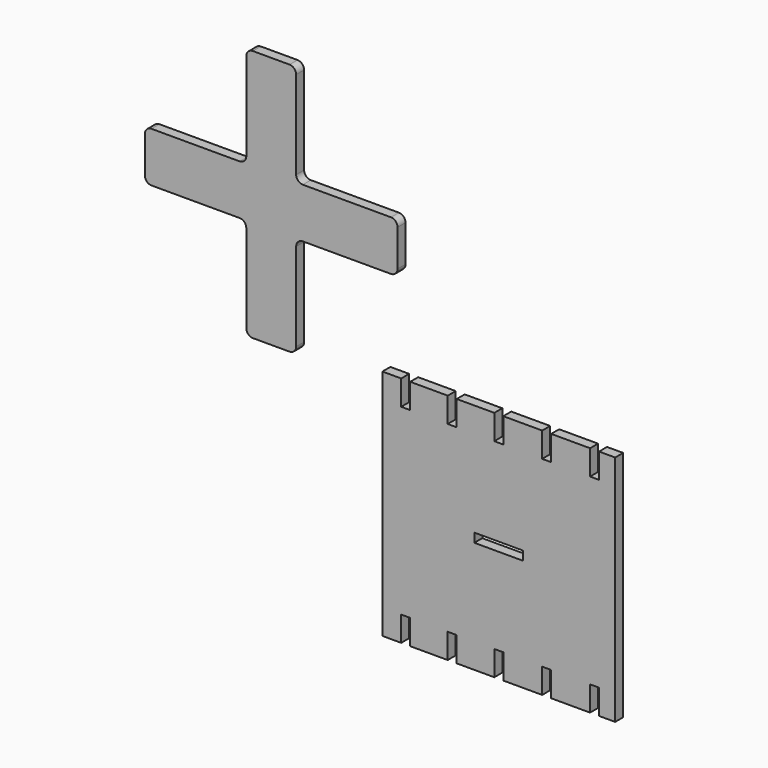
from build123d import *

# Parameters (mm, degrees)
F1_DEPTH = 3
F2_W     = 14.7
F2_H     = 2.7
F3_DEPTH = 3


# Not quite as in the source:
# - ends of sketch curves that miss each other by under 0.0002 mm in the source are joined


with BuildPart() as f1:
    # F0 (on Front) → F1 (new body)
    with BuildSketch(Plane.XZ):
        with BuildLine():
            ThreePointArc((-56.8837374449, 13.9543364197), (-56.2979510073, 12.5401228573), (-54.8837374449, 11.9543364197))
            Line((-54.8837374449, 11.9543364197), (-43.8837374449, 11.9543364197))
            ThreePointArc((-43.8837374449, 11.9543364197), (-42.4695238825, 12.5401228573), (-41.8837374449, 13.9543364197))
            Line((-41.8837374449, 13.9543364197), (-41.8837374449, 40.4543364197))
            ThreePointArc((-41.8837374449, 40.4543364197), (-41.2979510073, 41.8685499821), (-39.8837374449, 42.4543364197))
            Line((-39.8837374449, 42.4543364197), (-13.3837374449, 42.4543364197))
            ThreePointArc((-13.3837374449, 42.4543364197), (-11.9695238825, 43.0401228573), (-11.3837374449, 44.4543364197))
            Line((-11.3837374449, 44.4543364197), (-11.3837374449, 55.4543364197))
            ThreePointArc((-11.3837374449, 55.4543364197), (-11.9695238825, 56.8685499821), (-13.3837374449, 57.4543364197))
            Line((-13.3837374449, 57.4543364197), (-39.8837374449, 57.4543364197))
            ThreePointArc((-39.8837374449, 57.4543364197), (-41.2979510073, 58.0401228573), (-41.8837374449, 59.4543364197))
            Line((-41.8837374449, 59.4543364197), (-41.8837374449, 85.9543364197))
            ThreePointArc((-41.8837374449, 85.9543364197), (-42.4695238825, 87.3685499821), (-43.8837374449, 87.9543364197))
            Line((-43.8837374449, 87.9543364197), (-54.8837374449, 87.9543364197))
            ThreePointArc((-54.8837374449, 87.9543364197), (-56.2979510073, 87.3685499821), (-56.8837374449, 85.9543364197))
            Line((-56.8837374449, 85.9543364197), (-56.8837374449, 59.4543364197))
            ThreePointArc((-56.8837374449, 59.4543364197), (-57.4695238825, 58.0401228573), (-58.8837374449, 57.4543364197))
            Line((-58.8837374449, 57.4543364197), (-85.3837374449, 57.4543364197))
            ThreePointArc((-85.3837374449, 57.4543364197), (-86.7979532126, 56.8685499821), (-87.3837396502, 55.4543364197))
            Line((-87.3837396502, 55.4543364197), (-87.3837374449, 44.4543364197))
            ThreePointArc((-87.3837374449, 44.4543364197), (-86.7979510073, 43.0401228573), (-85.3837374449, 42.4543364197))
            Line((-85.3837374449, 42.4543364197), (-58.8837374449, 42.4543364197))
            ThreePointArc((-58.8837374449, 42.4543364197), (-57.4695238825, 41.8685499821), (-56.8837374449, 40.4543364197))
            Line((-56.8837374449, 40.4543364197), (-56.8837374449, 13.9543364197))
        make_face()
    extrude(amount=F1_DEPTH)


with BuildPart() as f3:
    # F2 (on Front) → F3 (new body)
    with BuildSketch(Plane.XZ):
        Polygon((54.0467553358, -54.2169875913), (54.0467553358, 15.7830124087), (49.1967553358, 15.7830124087), (49.1967553358, 8.2830124087), (46.4967553358, 8.2830124087), (46.4967553358, 15.7830124087), (34.7967553358, 15.7830124087), (34.7967553358, 8.2830124087), (32.0967553358, 8.2830124087), (32.0967553358, 15.7830124087), (20.3967553358, 15.7830124087), (20.3967553358, 8.2830124087), (17.6967553358, 8.2830124087), (17.6967553358, 15.7830124087), (6.3967553358, 15.7830124087), (6.3967553358, 8.2830124087), (3.6967553358, 8.2830124087), (3.6967553358, 15.7830124087), (-7.6032446642, 15.7830124087), (-7.6032446642, 8.2830124087), (-10.3032446642, 8.2830124087), (-10.3032446642, 15.7830124087), (-15.9532446642, 15.7830124087), (-15.9532446642, -54.2169875913), (-10.3032446642, -54.2169875913), (-10.3032446642, -46.7169875913), (-7.6032446642, -46.7169875913), (-7.6032446642, -54.2169875913), (3.6967553358, -54.2169875913), (3.6967553358, -46.7169875913), (6.3967553358, -46.7169875913), (6.3967553358, -54.2169875913), (17.6967553358, -54.2169875913), (17.6967553358, -46.7169875913), (20.3967553358, -46.7169875913), (20.3967553358, -54.2169875913), (32.0967553358, -54.2169875913), (32.0967553358, -46.7169875913), (34.7967553358, -46.7169875913), (34.7967553358, -54.2169875913), (46.4967553358, -54.2169875913), (46.4967553358, -46.7169875913), (49.1967553358, -46.7169875913), (49.1967553358, -54.2169875913), align=None)
        with Locations((19.0467553358, -19.2169875913)):
            Rectangle(F2_W, F2_H, mode=Mode.SUBTRACT)
    extrude(amount=F3_DEPTH)


solid = Compound([f1.part, f3.part])
